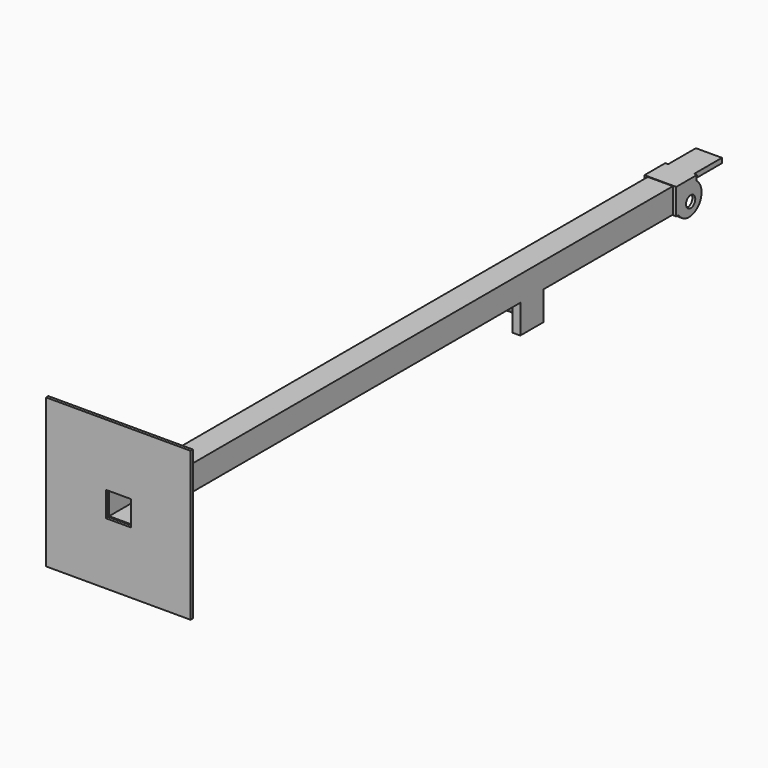
from build123d import *

# Parameters (mm, degrees)
F0_W      = 26
F0_H      = 26
F0_W_2    = 24
F0_H_2    = 24
F1_DEPTH  = 700
F2_W      = 27
F2_H      = 27
F2_W_2    = 26
F2_H_2    = 26
F2_W_3    = 24
F2_H_3    = 24
F3_DEPTH  = 3
F4_W      = 150
F4_H      = 154.387555053
F4_W_2    = 26
F4_H_2    = 26
F5_DEPTH  = 3
F6_W      = 27
F6_H      = 5
F7_DEPTH  = 65
F8_SIZE   = 4.99999
F10_DEPTH = 3
F12_DEPTH = 3
F14_D     = 12
F15_W     = 8
F15_H     = 30
F16_DEPTH = 30
F17_R     = 6.9361526391
F18_DEPTH = 35


# Not quite as in the source:
# - a fillet or chamfer is up to 0.001 mm smaller than in the source, because OpenCascade refuses the exact size


with BuildPart() as f1:
    # F0 (on Front) → F1 (new body)
    with BuildSketch(Plane.XZ):
        Rectangle(F0_W, F0_H)
        Rectangle(F0_W_2, F0_H_2, mode=Mode.SUBTRACT)
    extrude(amount=F1_DEPTH)

    # F2 (on face) → F3 (join)
    with BuildSketch(Plane(origin=(0, 0, 0), x_dir=(-1, 0, 0), z_dir=(0, 1, 0))):
        Rectangle(F2_W, F2_H)
        Rectangle(F2_W_2, F2_H_2, mode=Mode.SUBTRACT)
        Rectangle(F2_W_2, F2_H_2)
        Rectangle(F2_W_3, F2_H_3, mode=Mode.SUBTRACT)
        Rectangle(F2_W_3, F2_H_3)
    extrude(amount=F3_DEPTH)

    # F6 (on face) → F7 (join)
    with BuildSketch(Plane(origin=(0, 3, 0), x_dir=(-1, 0, 0), z_dir=(0, 1, 0))):
        with Locations((0, 11)):
            Rectangle(F6_W, F6_H)
    extrude(amount=F7_DEPTH)

    # F8 (size 5 in the source; OpenCascade refuses exactly that, so slightly less here)
    f8_edges = [f1.edges().sort_by_distance(p)[0] for p in [
        (13.5, 68, 11),
        (0, 68, 13.5),
        (-13.5, 68, 11),
    ]]
    chamfer(f8_edges, length=F8_SIZE)

    # F9 (on face) → F10 (join)
    with BuildSketch(Plane.YZ.offset(13.5)):
        Polygon((0, -13.5), (3, -13.5), (3, 8.5), (26.0593052953, 8.5), (26.8148947507, 13.5), (0, 13.5), align=None)
        with BuildLine():
            Line((3, 8.5), (3, -13.5))
            ThreePointArc((3, -13.5), (27.8075589796, -16.4172407177), (26.0593052953, 8.5))
            Line((26.0593052953, 8.5), (3, 8.5))
        make_face()
    extrude(amount=F10_DEPTH)

    # F11 (on face) → F12 (join)
    with BuildSketch(Plane(origin=(-13.5, 0, 0), x_dir=(0, -1, 0), z_dir=(-1, 0, 0))):
        Polygon((-27.0638596267, 13.5), (-25.7802139968, 8.5), (-3, 8.5), (-3, -13.5), (0, -13.5), (0, 13.5), align=None)
        with BuildLine():
            Line((-3, 8.5), (-25.7802139968, 8.5))
            ThreePointArc((-25.7802139968, 8.5), (-27.8924695055, -16.4812139716), (-3, -13.5))
            Line((-3, -13.5), (-3, 8.5))
        make_face()
    extrude(amount=F12_DEPTH)

    # F14 (through all)
    with Locations(Plane.YZ.offset(16.5)):
        with Locations((18.6792816967, -7.5708841905)):
            Hole(F14_D / 2)

    # F15 (on face) → F16 (join)
    with BuildSketch(Plane(origin=(0, 0, -13), x_dir=(1, 0, 0), z_dir=(0, 0, -1))):
        with Locations((9, 182.907372117)):
            Rectangle(F15_W, F15_H)
    extrude(amount=F16_DEPTH)

    # F17 (on face) → F18 (join)
    with BuildSketch(Plane(origin=(5, 0, 0), x_dir=(0, -1, 0), z_dir=(-1, 0, 0))):
        with Locations((182.907372117, -26.4493469149)):
            Circle(F17_R)
    extrude(amount=F18_DEPTH)


with BuildPart() as f5:
    # F4 (on face) → F5 (new body)
    with BuildSketch(Plane.XZ.offset(700)):
        Rectangle(F4_W, F4_H)
        Rectangle(F4_W_2, F4_H_2, mode=Mode.SUBTRACT)
    extrude(amount=F5_DEPTH)


solid = Compound([f1.part, f5.part])
